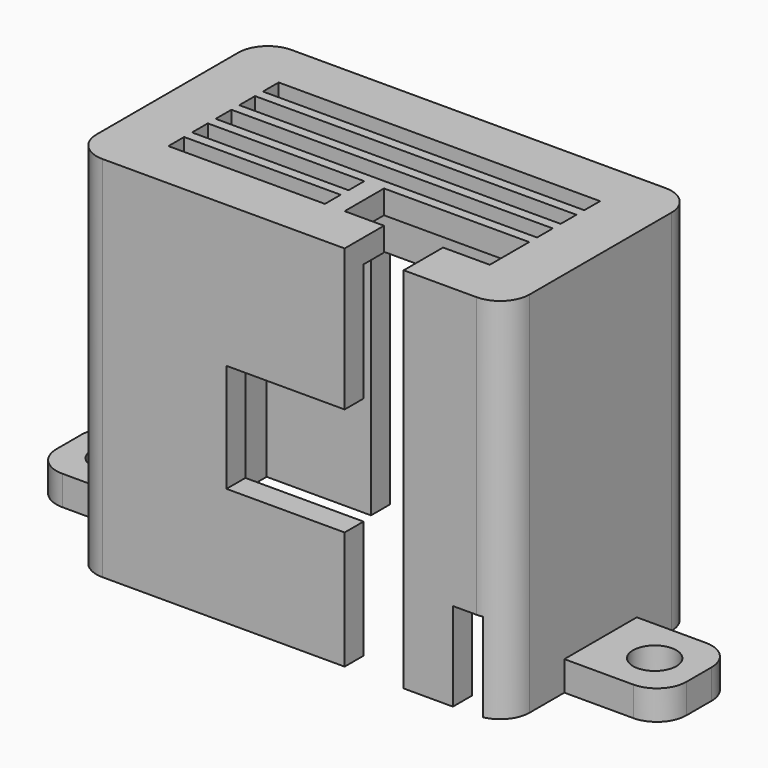
from build123d import *

# Parameters (mm, degrees)
F0_R      = 1.1
F1_DEPTH  = 1.5
F2_W      = 19.6000001132
F2_H      = 9.6000001132
F3_DEPTH  = 16
F4_W      = 1.5
F4_H      = 4.5
F4_W_2    = 6
F4_H_2    = 5.5
F5_DEPTH  = 1.2
F6_W      = 9
F6_H      = 12
F7_DEPTH  = 25
F8_W      = 16.3223941345
F8_H      = 1
F9_DEPTH  = 1.2
F10_W     = 3
F10_H     = 1.2
F11_DEPTH = 4
F12_W     = 3
F12_H     = 1
F12_W_2   = 2.3728397638
F13_DEPTH = 1.2
F14_W     = 2
F14_H     = 2.5
F14_W_2   = 2.3728397638
F15_DEPTH = 1.2


# Not quite as in the source:
# - a feature names something its author has since deleted; it is built from what else it names


with BuildPart() as f1:
    # F0 (on Top) → F1 (new body)
    with BuildSketch(Plane.XY):
        with BuildLine():
            Line((20.5, 0), (1.5, 0))
            ThreePointArc((1.5, 0), (0.4393398282, -0.4393398282), (0, -1.5))
            Line((0, -1.5), (0, -3.7))
            Line((0, -3.7), (0, -8.3))
            Line((0, -8.3), (0, -10.5))
            ThreePointArc((0, -10.5), (0.4393398282, -11.5606601718), (1.5, -12))
            Line((1.5, -12), (20.5, -12))
            ThreePointArc((20.5, -12), (21.5606601718, -11.5606601718), (22, -10.5))
            Line((22, -10.5), (22, -8.3))
            Line((22, -8.3), (22, -3.7))
            Line((22, -3.7), (22, -1.5))
            ThreePointArc((22, -1.5), (21.5606601718, -0.4393398282), (20.5, 0))
        make_face()
        Polygon((20.8000000566, -1.1999999434), (20.8000000566, -1.5), (20.8000000566, -10.5), (20.8000000566, -10.8000000566), (20.5, -10.8000000566), (1.5, -10.8000000566), (1.1999999434, -10.8000000566), (1.1999999434, -10.5), (1.1999999434, -1.5), (1.1999999434, -1.1999999434), (1.5, -1.1999999434), (20.5, -1.1999999434), align=None, mode=Mode.SUBTRACT)
        with BuildLine():
            Line((0, -8.3), (0, -3.7))
            Line((0, -3.7), (-3.5, -3.7))
            ThreePointArc((-3.5, -3.7), (-4.5606601718, -4.1393398282), (-5, -5.2))
            Line((-5, -5.2), (-5, -6.8))
            ThreePointArc((-5, -6.8), (-4.5606601718, -7.8606601718), (-3.5, -8.3))
            Line((-3.5, -8.3), (0, -8.3))
        make_face()
        with Locations((-2.75, -6)):
            Circle(F0_R, mode=Mode.SUBTRACT)
        with BuildLine():
            Line((25.5, -3.7), (22, -3.7))
            Line((22, -3.7), (22, -8.3))
            Line((22, -8.3), (25.5, -8.3))
            ThreePointArc((25.5, -8.3), (26.5606601718, -7.8606601718), (27, -6.8))
            Line((27, -6.8), (27, -5.2))
            ThreePointArc((27, -5.2), (26.5606601718, -4.1393398282), (25.5, -3.7))
        make_face()
        with Locations((24.75, -6)):
            Circle(F0_R, mode=Mode.SUBTRACT)
    extrude(amount=F1_DEPTH)

    # F2 (on face) → F3 (join)
    with BuildSketch(Plane.XY.offset(1.5)):
        with BuildLine():
            Line((22, -10.5), (22, -8.3))
            Line((22, -8.3), (22, -3.7))
            Line((22, -3.7), (22, -1.5))
            ThreePointArc((22, -1.5), (21.5606601718, -0.4393398282), (20.5, 0))
            Line((20.5, 0), (1.5, 0))
            ThreePointArc((1.5, 0), (0.4393398282, -0.4393398282), (0, -1.5))
            Line((0, -1.5), (0, -3.7))
            Line((0, -3.7), (0, -8.3))
            Line((0, -8.3), (0, -10.5))
            ThreePointArc((0, -10.5), (0.4393398282, -11.5606601718), (1.5, -12))
            Line((1.5, -12), (20.5, -12))
            ThreePointArc((20.5, -12), (21.5606601718, -11.5606601718), (22, -10.5))
        make_face()
        with Locations((11, -6)):
            Rectangle(F2_W, F2_H, mode=Mode.SUBTRACT)
    extrude(amount=F3_DEPTH)

    # F4 (on face) → F5 (cut)
    with BuildSketch(Plane(origin=(0, -10.8000000566, 0), x_dir=(-1, 0, 0), z_dir=(0, 1, 0))):
        with Locations((-20.0500000566, 2.25)):
            Rectangle(F4_W, F4_H)
        Polygon((-16.8000000566, 17.5), (-16.8000000566, 0), (-13.8000000566, 0), (-13.8000000566, 6), (-13.8000000566, 11.5), (-13.8000000566, 17.5), align=None)
        with Locations((-10.8000000566, 8.75)):
            Rectangle(F4_W_2, F4_H_2)
    extrude(amount=-F5_DEPTH, mode=Mode.SUBTRACT)

    # F6 (on face) → F7 (cut)
    with BuildSketch(Plane.XZ.offset(1.1999999434)):
        with Locations((10.9999999434, 6)):
            Rectangle(F6_W, F6_H)
    extrude(amount=-F7_DEPTH, mode=Mode.SUBTRACT)

    # F8 (on face) → F9 (join)
    with BuildSketch(Plane.XY.offset(17.5)):
        with BuildLine():
            Line((16.8000000566, -10.8000000566), (16.8000000566, -12.0000000566))
            Line((16.8000000566, -12), (20.5, -12))
            ThreePointArc((20.5, -12), (21.5606601718, -11.5606601718), (22, -10.5))
            Line((22, -10.5), (22, -1.5))
            ThreePointArc((22, -1.5), (21.5606601718, -0.4393398282), (20.5, 0))
            Line((20.5, 0), (1.5, 0))
            ThreePointArc((1.5, 0), (0.4393398282, -0.4393398282), (0, -1.5))
            Line((0, -1.5), (0, -10.5))
            ThreePointArc((0, -10.5), (0.4393398282, -11.5606601718), (1.5, -12))
            Line((1.5, -12), (13.8000000566, -12))
            Line((13.8000000566, -12.0000000566), (13.8000000566, -10.8000000566))
            Line((13.8000000566, -10.8000000566), (1.1999999434, -10.8000000566))
            Line((1.1999999434, -10.8000000566), (1.1999999434, -1.1999999434))
            Line((1.1999999434, -1.1999999434), (20.8000000566, -1.1999999434))
            Line((20.8000000566, -1.1999999434), (20.8000000566, -10.8000000566))
            Line((20.8000000566, -10.8000000566), (16.8000000566, -10.8000000566))
        make_face()
        Polygon((13.8000000566, -12), (16.8000000566, -12), (16.8000000566, -10.8000000566), (20.8000000566, -10.8000000566), (20.8000000566, -1.1999999434), (1.1999999434, -1.1999999434), (1.1999999434, -10.8000000566), (13.8000000566, -10.8000000566), align=None)
        with Locations((11.0116427531, -9)):
            Rectangle(F8_W, F8_H, mode=Mode.SUBTRACT)
        with Locations((11.0116427531, -7.5)):
            Rectangle(F8_W, F8_H, mode=Mode.SUBTRACT)
        with Locations((11.0116427531, -6)):
            Rectangle(F8_W, F8_H, mode=Mode.SUBTRACT)
        with Locations((11.0116427531, -4.5)):
            Rectangle(F8_W, F8_H, mode=Mode.SUBTRACT)
        with Locations((11.0116427531, -3)):
            Rectangle(F8_W, F8_H, mode=Mode.SUBTRACT)
    extrude(amount=F9_DEPTH)

    # F10 (on face) → F11 (cut)
    with BuildSketch(Plane.XZ.offset(12)):
        with Locations((15.3000000566, 18.1)):
            Rectangle(F10_W, F10_H)
    extrude(amount=-F11_DEPTH, mode=Mode.SUBTRACT)

    # F12 (on face) → F13 (join)
    with BuildSketch(Plane.XY.offset(18.7)):
        with Locations((12.3000000566, -9)):
            Rectangle(F12_W, F12_H)
        with Locations((12.3000000566, -7.5)):
            Rectangle(F12_W, F12_H)
        with Locations((17.9864199385, -7.5)):
            Rectangle(F12_W_2, F12_H)
        with Locations((17.9864199385, -9)):
            Rectangle(F12_W_2, F12_H)
    extrude(amount=-F13_DEPTH)

    # F14 (on face) → F15 (cut)
    with BuildSketch(Plane.XY.offset(18.7)):
        with Locations((12.8000000566, -8.25)):
            Rectangle(F14_W, F14_H)
        with Locations((17.9864199385, -8.25)):
            Rectangle(F14_W_2, F14_H)
    extrude(amount=-F15_DEPTH, mode=Mode.SUBTRACT)


solid = f1.part
